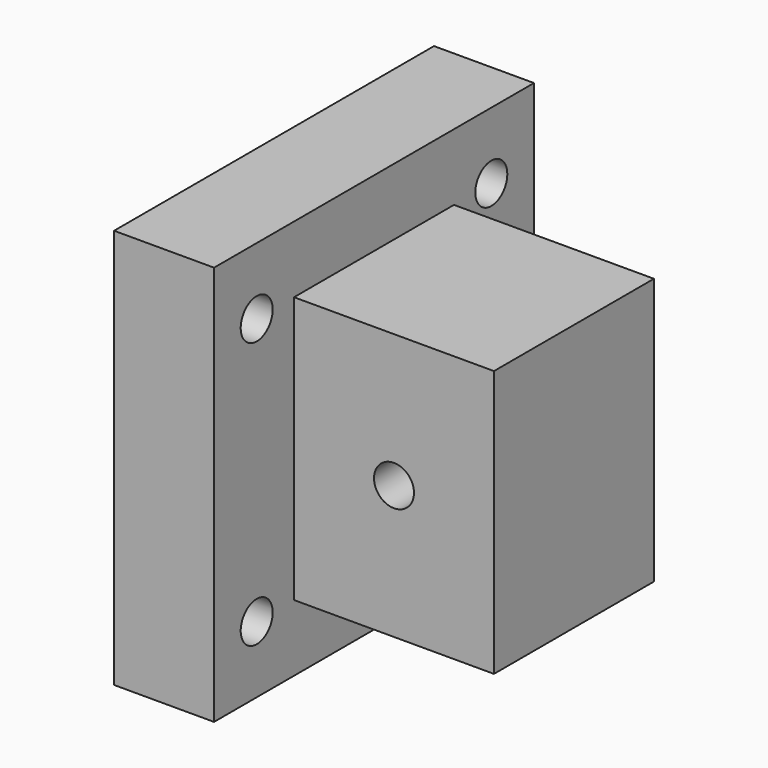
from build123d import *

# Parameters (mm, degrees)
F0_W     = 60
F0_H     = 60
F0_R     = 3
F0_W_2   = 30
F0_H_2   = 40
F1_DEPTH = 15
F2_DEPTH = 30
F3_R     = 3
F4_DEPTH = 45.001


# Not quite as in the source:
# - a feature names something its author has since deleted; it is built from what else it names


with BuildPart() as f1:
    # F0 (on Right) → F1 (new body)
    with BuildSketch(Plane.YZ):
        Rectangle(F0_W, F0_H)
        with Locations((-22, -20)):
            Circle(F0_R, mode=Mode.SUBTRACT)
        with Locations((22, -20)):
            Circle(F0_R, mode=Mode.SUBTRACT)
        with Locations((-22, 20)):
            Circle(F0_R, mode=Mode.SUBTRACT)
        Rectangle(F0_W_2, F0_H_2, mode=Mode.SUBTRACT)
        with Locations((22, 20)):
            Circle(F0_R, mode=Mode.SUBTRACT)
        Rectangle(F0_W_2, F0_H_2)
    extrude(amount=-F1_DEPTH)

    # F0 (on Right) → F2 (join)
    with BuildSketch(Plane.YZ):
        Rectangle(F0_W_2, F0_H_2)
    extrude(amount=F2_DEPTH)

    # F3 (on face) → F4 (cut, through all)
    with BuildSketch(Plane.XZ.offset(15)):
        with Locations((15, 0)):
            Circle(F3_R)
    extrude(amount=-F4_DEPTH, mode=Mode.SUBTRACT)


solid = f1.part
